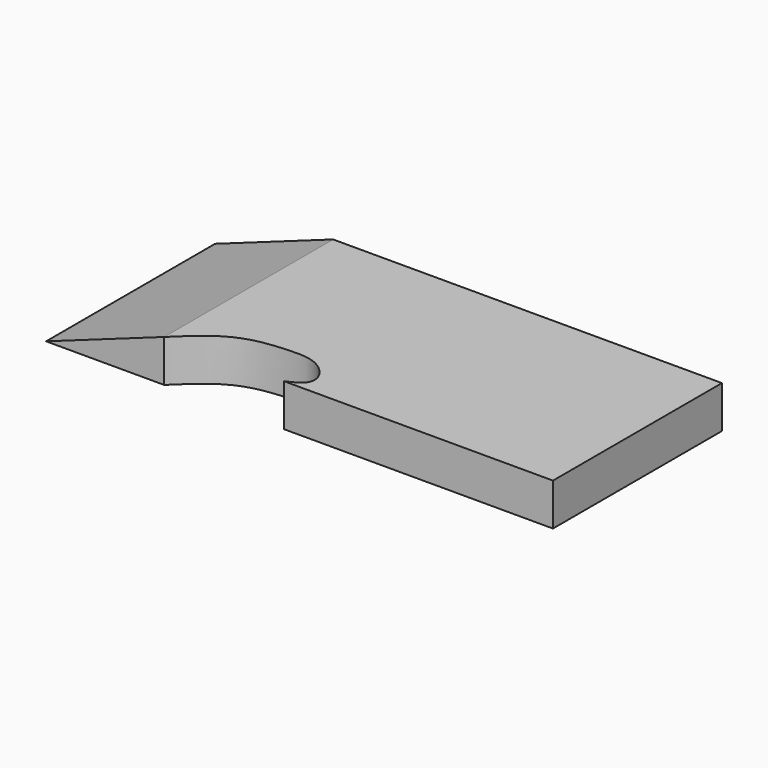
from build123d import *

# Parameters (mm, degrees)
F1_DEPTH = 6.35
F2_SIZE2 = 6.34999
F2_SIZE  = 17.75459


# Not quite as in the source:
# - a fillet or chamfer is up to 0.001 mm smaller than in the source, because OpenCascade refuses the exact size


with BuildPart() as f1:
    # F0 (on Top) → F1 (new body)
    with BuildSketch(Plane.XY):
        with BuildLine():
            Line((38.1, 15.875), (-38.1, 15.875))
            Line((-38.1, 15.875), (-38.1, -15.875))
            Line((-38.1, -15.875), (-20.3513801098, -15.875))
            add(Edge.make_bspline(
                [(-20.3513801098, -15.875), (-19.5442600635, -15.0806070794), (-17.8938059161, -13.4561782272), (-14.8392122853, -11.1202028199), (-11.2582679077, -9.7102875395), (-6.2422908773, -9.2564413312), (-2.450482189, -9.4578887631), (0.3163590299, -12.0282683935), (0.3966126589, -14.6462649088), (-1.3919718956, -15.4452723731), (-2.3539206013, -15.875)],
                knots=[0, 0, 0, 0, 0.1245260011, 0.2546392645, 0.3863068952, 0.5364470911, 0.6667795698, 0.7909479354, 0.8875661973, 1, 1, 1, 1], degree=3))
            Line((-2.3539206013, -15.875), (38.1, -15.875))
            Line((38.1, -15.875), (38.1, 15.875))
        make_face()
    extrude(amount=F1_DEPTH)

    # F2 (size 17.7546 and 6.35 in the source; OpenCascade refuses exactly that, so slightly less here)
    f2_edges = [f1.edges().sort_by_distance(p)[0] for p in [
        (-38.1, 0, 6.35),
    ]]
    f2_side = f1.faces().sort_by_distance((0.37676, 0.562053, 6.35))[0]
    chamfer(f2_edges, length=F2_SIZE, length2=F2_SIZE2, reference=f2_side)


solid = f1.part
